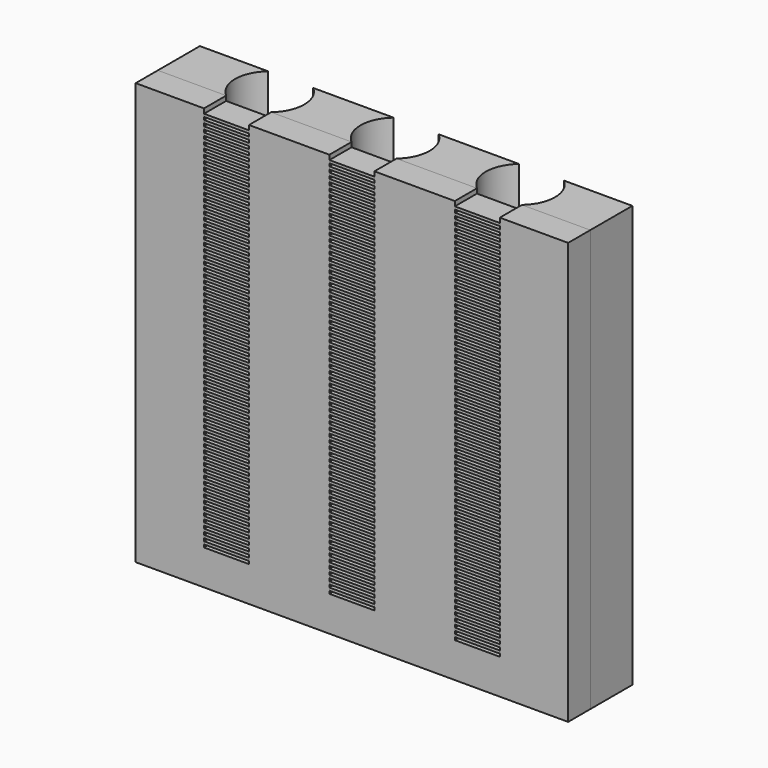
from build123d import *

# Parameters (mm, degrees)
F0_W         = 78.14
F0_H         = 9.5
F1_DEPTH     = 76.2
F2_R         = 6.25
F3_DEPTH     = 69.85
F4_TEXT_SIZE = 6.2920652474
F5_DEPTH     = 1
F6_W         = 8.1240384046
F6_H         = 0.5
F7_DEPTH     = 5
F9_DEPTH     = 5


# Not quite as in the source:
# - Text() gives the source's letters only with a copy of the font that has no kerning and outlines rounded to 1/6400 em; it was checked with that copy


with BuildPart() as f1:
    # F0 (on Top) → F1 (new body)
    with BuildSketch(Plane.XY):
        Rectangle(F0_W, F0_H)
    extrude(amount=F1_DEPTH)

    # F2 (on face) → F3 (cut)
    with BuildSketch(Plane.XY.offset(76.2)):
        with Locations((-22.66, 0)):
            Circle(F2_R)
        Circle(F2_R)
        with Locations((22.66, 0)):
            Circle(F2_R)
    extrude(amount=-F3_DEPTH, mode=Mode.SUBTRACT)

    # F4 (on face) → F5 (cut)
    with BuildSketch(Plane.XZ.offset(4.75)):
        with Locations((-26.469767316, 1.2358349282)):
            Text('1            2              3', F4_TEXT_SIZE, font='Open Sans', text_align=(TextAlign.LEFT, TextAlign.BOTTOM))
    extrude(amount=-F5_DEPTH, mode=Mode.SUBTRACT)


with BuildPart() as f7:
    # F6 (on face) → F7 (new body)
    with BuildSketch(Plane.XZ.offset(4.75)):
        with Locations((-22.66, 7.1)):
            Rectangle(F6_W, F6_H)
        with Locations((-22.66, 8.1)):
            Rectangle(F6_W, F6_H)
        with Locations((-22.66, 9.1)):
            Rectangle(F6_W, F6_H)
        with Locations((-22.66, 10.1)):
            Rectangle(F6_W, F6_H)
        with Locations((-22.66, 11.1)):
            Rectangle(F6_W, F6_H)
        with Locations((-22.66, 12.1)):
            Rectangle(F6_W, F6_H)
        with Locations((-22.66, 13.1)):
            Rectangle(F6_W, F6_H)
        with Locations((-22.66, 14.1)):
            Rectangle(F6_W, F6_H)
        with Locations((-22.66, 15.1)):
            Rectangle(F6_W, F6_H)
        with Locations((-22.66, 16.1)):
            Rectangle(F6_W, F6_H)
        with Locations((-22.66, 17.1)):
            Rectangle(F6_W, F6_H)
        with Locations((-22.66, 18.1)):
            Rectangle(F6_W, F6_H)
        with Locations((-22.66, 19.1)):
            Rectangle(F6_W, F6_H)
        with Locations((-22.66, 20.1)):
            Rectangle(F6_W, F6_H)
        with Locations((-22.66, 21.1)):
            Rectangle(F6_W, F6_H)
        with Locations((-22.66, 22.1)):
            Rectangle(F6_W, F6_H)
        with Locations((-22.66, 23.1)):
            Rectangle(F6_W, F6_H)
        with Locations((-22.66, 24.1)):
            Rectangle(F6_W, F6_H)
        with Locations((-22.66, 25.1)):
            Rectangle(F6_W, F6_H)
        with Locations((-22.66, 26.1)):
            Rectangle(F6_W, F6_H)
        with Locations((-22.66, 27.1)):
            Rectangle(F6_W, F6_H)
        with Locations((-22.66, 28.1)):
            Rectangle(F6_W, F6_H)
        with Locations((-22.66, 29.1)):
            Rectangle(F6_W, F6_H)
        with Locations((-22.66, 30.1)):
            Rectangle(F6_W, F6_H)
        with Locations((-22.66, 31.1)):
            Rectangle(F6_W, F6_H)
        with Locations((-22.66, 32.1)):
            Rectangle(F6_W, F6_H)
        with Locations((-22.66, 33.1)):
            Rectangle(F6_W, F6_H)
        with Locations((-22.66, 34.1)):
            Rectangle(F6_W, F6_H)
        with Locations((-22.66, 35.1)):
            Rectangle(F6_W, F6_H)
        with Locations((-22.66, 36.1)):
            Rectangle(F6_W, F6_H)
        with Locations((-22.66, 37.1)):
            Rectangle(F6_W, F6_H)
        with Locations((-22.66, 38.1)):
            Rectangle(F6_W, F6_H)
        with Locations((-22.66, 39.1)):
            Rectangle(F6_W, F6_H)
        with Locations((-22.66, 40.1)):
            Rectangle(F6_W, F6_H)
        with Locations((-22.66, 41.1)):
            Rectangle(F6_W, F6_H)
        with Locations((-22.66, 42.1)):
            Rectangle(F6_W, F6_H)
        with Locations((-22.66, 43.1)):
            Rectangle(F6_W, F6_H)
        with Locations((-22.66, 44.1)):
            Rectangle(F6_W, F6_H)
        with Locations((-22.66, 45.1)):
            Rectangle(F6_W, F6_H)
        with Locations((-22.66, 46.1)):
            Rectangle(F6_W, F6_H)
        with Locations((-22.66, 47.1)):
            Rectangle(F6_W, F6_H)
        with Locations((-22.66, 48.1)):
            Rectangle(F6_W, F6_H)
        with Locations((-22.66, 49.1)):
            Rectangle(F6_W, F6_H)
        with Locations((-22.66, 50.1)):
            Rectangle(F6_W, F6_H)
        with Locations((-22.66, 51.1)):
            Rectangle(F6_W, F6_H)
        with Locations((-22.66, 52.1)):
            Rectangle(F6_W, F6_H)
        with Locations((-22.66, 53.1)):
            Rectangle(F6_W, F6_H)
        with Locations((-22.66, 54.1)):
            Rectangle(F6_W, F6_H)
        with Locations((-22.66, 55.1)):
            Rectangle(F6_W, F6_H)
        with Locations((-22.66, 56.1)):
            Rectangle(F6_W, F6_H)
        with Locations((-22.66, 57.1)):
            Rectangle(F6_W, F6_H)
        with Locations((-22.66, 58.1)):
            Rectangle(F6_W, F6_H)
        with Locations((-22.66, 59.1)):
            Rectangle(F6_W, F6_H)
        with Locations((-22.66, 60.1)):
            Rectangle(F6_W, F6_H)
        with Locations((-22.66, 61.1)):
            Rectangle(F6_W, F6_H)
        with Locations((-22.66, 62.1)):
            Rectangle(F6_W, F6_H)
        with Locations((-22.66, 63.1)):
            Rectangle(F6_W, F6_H)
        with Locations((-22.66, 64.1)):
            Rectangle(F6_W, F6_H)
        with Locations((-22.66, 65.1)):
            Rectangle(F6_W, F6_H)
        with Locations((-22.66, 66.1)):
            Rectangle(F6_W, F6_H)
        with Locations((-22.66, 67.1)):
            Rectangle(F6_W, F6_H)
        with Locations((-22.66, 68.1)):
            Rectangle(F6_W, F6_H)
        with Locations((-22.66, 69.1)):
            Rectangle(F6_W, F6_H)
        with Locations((-22.66, 70.1)):
            Rectangle(F6_W, F6_H)
        with Locations((-22.66, 71.1)):
            Rectangle(F6_W, F6_H)
        with Locations((-22.66, 72.1)):
            Rectangle(F6_W, F6_H)
        with Locations((-22.66, 73.1)):
            Rectangle(F6_W, F6_H)
        with Locations((-22.66, 74.1)):
            Rectangle(F6_W, F6_H)
        with Locations((-22.66, 75.1)):
            Rectangle(F6_W, F6_H)
        with Locations((4e-07, 7.1)):
            Rectangle(F6_W, F6_H)
        with Locations((4e-07, 8.1)):
            Rectangle(F6_W, F6_H)
        with Locations((4e-07, 9.1)):
            Rectangle(F6_W, F6_H)
        with Locations((4e-07, 10.1)):
            Rectangle(F6_W, F6_H)
        with Locations((4e-07, 11.1)):
            Rectangle(F6_W, F6_H)
        with Locations((4e-07, 12.1)):
            Rectangle(F6_W, F6_H)
        with Locations((4e-07, 13.1)):
            Rectangle(F6_W, F6_H)
        with Locations((4e-07, 14.1)):
            Rectangle(F6_W, F6_H)
        with Locations((4e-07, 15.1)):
            Rectangle(F6_W, F6_H)
        with Locations((4e-07, 16.1)):
            Rectangle(F6_W, F6_H)
        with Locations((4e-07, 17.1)):
            Rectangle(F6_W, F6_H)
        with Locations((4e-07, 18.1)):
            Rectangle(F6_W, F6_H)
        with Locations((4e-07, 19.1)):
            Rectangle(F6_W, F6_H)
        with Locations((4e-07, 20.1)):
            Rectangle(F6_W, F6_H)
        with Locations((4e-07, 21.1)):
            Rectangle(F6_W, F6_H)
        with Locations((4e-07, 22.1)):
            Rectangle(F6_W, F6_H)
        with Locations((4e-07, 23.1)):
            Rectangle(F6_W, F6_H)
        with Locations((4e-07, 24.1)):
            Rectangle(F6_W, F6_H)
        with Locations((4e-07, 25.1)):
            Rectangle(F6_W, F6_H)
        with Locations((4e-07, 26.1)):
            Rectangle(F6_W, F6_H)
        with Locations((4e-07, 27.1)):
            Rectangle(F6_W, F6_H)
        with Locations((4e-07, 28.1)):
            Rectangle(F6_W, F6_H)
        with Locations((4e-07, 29.1)):
            Rectangle(F6_W, F6_H)
        with Locations((4e-07, 30.1)):
            Rectangle(F6_W, F6_H)
        with Locations((4e-07, 31.1)):
            Rectangle(F6_W, F6_H)
        with Locations((4e-07, 32.1)):
            Rectangle(F6_W, F6_H)
        with Locations((4e-07, 33.1)):
            Rectangle(F6_W, F6_H)
        with Locations((4e-07, 34.1)):
            Rectangle(F6_W, F6_H)
        with Locations((4e-07, 35.1)):
            Rectangle(F6_W, F6_H)
        with Locations((4e-07, 36.1)):
            Rectangle(F6_W, F6_H)
        with Locations((4e-07, 37.1)):
            Rectangle(F6_W, F6_H)
        with Locations((4e-07, 38.1)):
            Rectangle(F6_W, F6_H)
        with Locations((4e-07, 39.1)):
            Rectangle(F6_W, F6_H)
        with Locations((4e-07, 40.1)):
            Rectangle(F6_W, F6_H)
        with Locations((4e-07, 41.1)):
            Rectangle(F6_W, F6_H)
        with Locations((4e-07, 42.1)):
            Rectangle(F6_W, F6_H)
        with Locations((4e-07, 43.1)):
            Rectangle(F6_W, F6_H)
        with Locations((4e-07, 44.1)):
            Rectangle(F6_W, F6_H)
        with Locations((4e-07, 45.1)):
            Rectangle(F6_W, F6_H)
        with Locations((4e-07, 46.1)):
            Rectangle(F6_W, F6_H)
        with Locations((4e-07, 47.1)):
            Rectangle(F6_W, F6_H)
        with Locations((4e-07, 48.1)):
            Rectangle(F6_W, F6_H)
        with Locations((4e-07, 49.1)):
            Rectangle(F6_W, F6_H)
        with Locations((4e-07, 50.1)):
            Rectangle(F6_W, F6_H)
        with Locations((4e-07, 51.1)):
            Rectangle(F6_W, F6_H)
        with Locations((4e-07, 52.1)):
            Rectangle(F6_W, F6_H)
        with Locations((4e-07, 53.1)):
            Rectangle(F6_W, F6_H)
        with Locations((4e-07, 54.1)):
            Rectangle(F6_W, F6_H)
        with Locations((4e-07, 55.1)):
            Rectangle(F6_W, F6_H)
        with Locations((4e-07, 56.1)):
            Rectangle(F6_W, F6_H)
        with Locations((4e-07, 57.1)):
            Rectangle(F6_W, F6_H)
        with Locations((4e-07, 58.1)):
            Rectangle(F6_W, F6_H)
        with Locations((4e-07, 59.1)):
            Rectangle(F6_W, F6_H)
        with Locations((4e-07, 60.1)):
            Rectangle(F6_W, F6_H)
        with Locations((4e-07, 61.1)):
            Rectangle(F6_W, F6_H)
        with Locations((4e-07, 62.1)):
            Rectangle(F6_W, F6_H)
        with Locations((4e-07, 63.1)):
            Rectangle(F6_W, F6_H)
        with Locations((4e-07, 64.1)):
            Rectangle(F6_W, F6_H)
        with Locations((4e-07, 65.1)):
            Rectangle(F6_W, F6_H)
        with Locations((4e-07, 66.1)):
            Rectangle(F6_W, F6_H)
        with Locations((4e-07, 67.1)):
            Rectangle(F6_W, F6_H)
        with Locations((4e-07, 68.1)):
            Rectangle(F6_W, F6_H)
        with Locations((4e-07, 69.1)):
            Rectangle(F6_W, F6_H)
        with Locations((4e-07, 70.1)):
            Rectangle(F6_W, F6_H)
        with Locations((4e-07, 71.1)):
            Rectangle(F6_W, F6_H)
        with Locations((4e-07, 72.1)):
            Rectangle(F6_W, F6_H)
        with Locations((4e-07, 73.1)):
            Rectangle(F6_W, F6_H)
        with Locations((4e-07, 74.1)):
            Rectangle(F6_W, F6_H)
        with Locations((4e-07, 75.1)):
            Rectangle(F6_W, F6_H)
        with Locations((22.6600008, 7.1)):
            Rectangle(F6_W, F6_H)
        with Locations((22.6600008, 8.1)):
            Rectangle(F6_W, F6_H)
        with Locations((22.6600008, 9.1)):
            Rectangle(F6_W, F6_H)
        with Locations((22.6600008, 10.1)):
            Rectangle(F6_W, F6_H)
        with Locations((22.6600008, 11.1)):
            Rectangle(F6_W, F6_H)
        with Locations((22.6600008, 12.1)):
            Rectangle(F6_W, F6_H)
        with Locations((22.6600008, 13.1)):
            Rectangle(F6_W, F6_H)
        with Locations((22.6600008, 14.1)):
            Rectangle(F6_W, F6_H)
        with Locations((22.6600008, 15.1)):
            Rectangle(F6_W, F6_H)
        with Locations((22.6600008, 16.1)):
            Rectangle(F6_W, F6_H)
        with Locations((22.6600008, 17.1)):
            Rectangle(F6_W, F6_H)
        with Locations((22.6600008, 18.1)):
            Rectangle(F6_W, F6_H)
        with Locations((22.6600008, 19.1)):
            Rectangle(F6_W, F6_H)
        with Locations((22.6600008, 20.1)):
            Rectangle(F6_W, F6_H)
        with Locations((22.6600008, 21.1)):
            Rectangle(F6_W, F6_H)
        with Locations((22.6600008, 22.1)):
            Rectangle(F6_W, F6_H)
        with Locations((22.6600008, 23.1)):
            Rectangle(F6_W, F6_H)
        with Locations((22.6600008, 24.1)):
            Rectangle(F6_W, F6_H)
        with Locations((22.6600008, 25.1)):
            Rectangle(F6_W, F6_H)
        with Locations((22.6600008, 26.1)):
            Rectangle(F6_W, F6_H)
        with Locations((22.6600008, 27.1)):
            Rectangle(F6_W, F6_H)
        with Locations((22.6600008, 28.1)):
            Rectangle(F6_W, F6_H)
        with Locations((22.6600008, 29.1)):
            Rectangle(F6_W, F6_H)
        with Locations((22.6600008, 30.1)):
            Rectangle(F6_W, F6_H)
        with Locations((22.6600008, 31.1)):
            Rectangle(F6_W, F6_H)
        with Locations((22.6600008, 32.1)):
            Rectangle(F6_W, F6_H)
        with Locations((22.6600008, 33.1)):
            Rectangle(F6_W, F6_H)
        with Locations((22.6600008, 34.1)):
            Rectangle(F6_W, F6_H)
        with Locations((22.6600008, 35.1)):
            Rectangle(F6_W, F6_H)
        with Locations((22.6600008, 36.1)):
            Rectangle(F6_W, F6_H)
        with Locations((22.6600008, 37.1)):
            Rectangle(F6_W, F6_H)
        with Locations((22.6600008, 38.1)):
            Rectangle(F6_W, F6_H)
        with Locations((22.6600008, 39.1)):
            Rectangle(F6_W, F6_H)
        with Locations((22.6600008, 40.1)):
            Rectangle(F6_W, F6_H)
        with Locations((22.6600008, 41.1)):
            Rectangle(F6_W, F6_H)
        with Locations((22.6600008, 42.1)):
            Rectangle(F6_W, F6_H)
        with Locations((22.6600008, 43.1)):
            Rectangle(F6_W, F6_H)
        with Locations((22.6600008, 44.1)):
            Rectangle(F6_W, F6_H)
        with Locations((22.6600008, 45.1)):
            Rectangle(F6_W, F6_H)
        with Locations((22.6600008, 46.1)):
            Rectangle(F6_W, F6_H)
        with Locations((22.6600008, 47.1)):
            Rectangle(F6_W, F6_H)
        with Locations((22.6600008, 48.1)):
            Rectangle(F6_W, F6_H)
        with Locations((22.6600008, 49.1)):
            Rectangle(F6_W, F6_H)
        with Locations((22.6600008, 50.1)):
            Rectangle(F6_W, F6_H)
        with Locations((22.6600008, 51.1)):
            Rectangle(F6_W, F6_H)
        with Locations((22.6600008, 52.1)):
            Rectangle(F6_W, F6_H)
        with Locations((22.6600008, 53.1)):
            Rectangle(F6_W, F6_H)
        with Locations((22.6600008, 54.1)):
            Rectangle(F6_W, F6_H)
        with Locations((22.6600008, 55.1)):
            Rectangle(F6_W, F6_H)
        with Locations((22.6600008, 56.1)):
            Rectangle(F6_W, F6_H)
        with Locations((22.6600008, 57.1)):
            Rectangle(F6_W, F6_H)
        with Locations((22.6600008, 58.1)):
            Rectangle(F6_W, F6_H)
        with Locations((22.6600008, 59.1)):
            Rectangle(F6_W, F6_H)
        with Locations((22.6600008, 60.1)):
            Rectangle(F6_W, F6_H)
        with Locations((22.6600008, 61.1)):
            Rectangle(F6_W, F6_H)
        with Locations((22.6600008, 62.1)):
            Rectangle(F6_W, F6_H)
        with Locations((22.6600008, 63.1)):
            Rectangle(F6_W, F6_H)
        with Locations((22.6600008, 64.1)):
            Rectangle(F6_W, F6_H)
        with Locations((22.6600008, 65.1)):
            Rectangle(F6_W, F6_H)
        with Locations((22.6600008, 66.1)):
            Rectangle(F6_W, F6_H)
        with Locations((22.6600008, 67.1)):
            Rectangle(F6_W, F6_H)
        with Locations((22.6600008, 68.1)):
            Rectangle(F6_W, F6_H)
        with Locations((22.6600008, 69.1)):
            Rectangle(F6_W, F6_H)
        with Locations((22.6600008, 70.1)):
            Rectangle(F6_W, F6_H)
        with Locations((22.6600008, 71.1)):
            Rectangle(F6_W, F6_H)
        with Locations((22.6600008, 72.1)):
            Rectangle(F6_W, F6_H)
        with Locations((22.6600008, 73.1)):
            Rectangle(F6_W, F6_H)
        with Locations((22.6600008, 74.1)):
            Rectangle(F6_W, F6_H)
        with Locations((22.6600008, 75.1)):
            Rectangle(F6_W, F6_H)
    extrude(amount=F7_DEPTH)


with BuildPart() as f9:
    # F8 (on face) → F9 (new body)
    with BuildSketch(Plane.XZ.offset(4.75)):
        Polygon((-26.7220192023, 76.2), (-39.07, 76.2), (-39.07, 0), (39.07, 0), (39.07, 76.2), (26.7220192023, 76.2), (26.7220192023, 6.35), (18.5979807977, 6.35), (18.5979807977, 76.2), (4.0620192023, 76.2), (4.0620192023, 6.35), (-4.0620192023, 6.35), (-4.0620192023, 76.2), (-18.5979807977, 76.2), (-18.5979807977, 6.35), (-26.7220192023, 6.35), align=None)
    extrude(amount=F9_DEPTH)


solid = Compound([f1.part, f7.part, f9.part])
